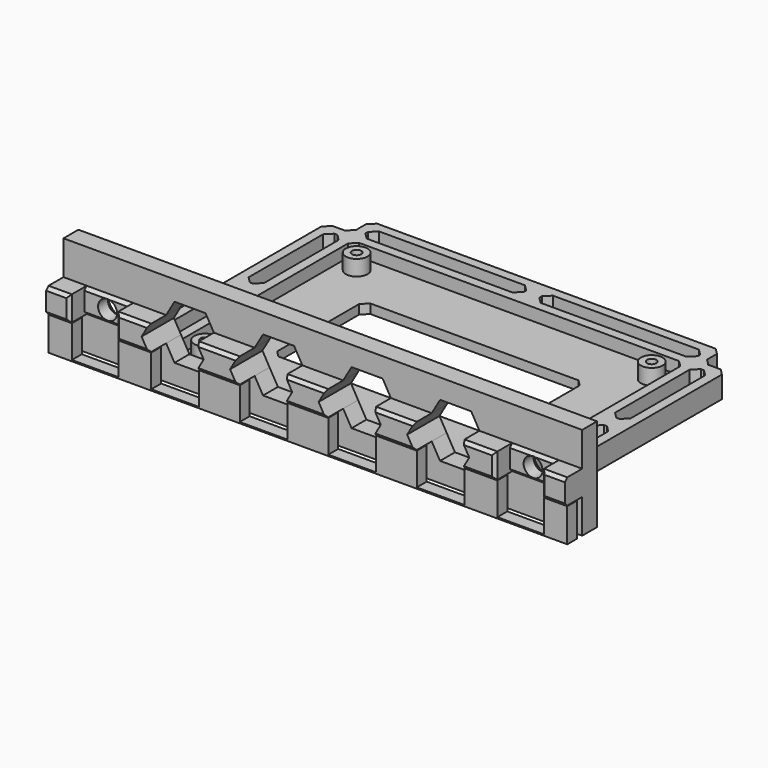
from build123d import *

# Parameters (mm, degrees)
F0_W          = 107
F0_H          = 73
F0_R          = 3.5
F0_W_2        = 71
F0_H_2        = 37
F0_R_2        = 1.5
F0_W_3        = 5
F0_H_3        = 5
F0_W_4        = 3
F0_H_4        = 3
F1_DEPTH      = 3
F2_DEPTH      = 4
F3_DEPTH      = 5
F4_DEPTH      = 27
F5_R          = 3.05
F6_DEPTH      = 6
F7_DEPTH      = 3
F5_W          = 7.5
F5_H          = 8
F8_DEPTH      = 7
F9_DEPTH      = 1
F10_T1_DEPTH  = 12.6433659759
F10_T3_DEPTH  = 15.7027670527
F10_T5_DEPTH  = 18.2621681294
F10_T7_DEPTH  = 18.2621681294
F10_T9_DEPTH  = 18.2621681294
F10_T11_DEPTH = 15.7027670527
F10_T13_DEPTH = 12.6433659759
F10_T15_DEPTH = 13.1433659759
F10_T20_DEPTH = 15
F10_T25_DEPTH = 15
F10_T30_DEPTH = 15
F10_T35_DEPTH = 15
F11_SIZE      = 2
F12_W         = 7.5
F12_H         = 4
F12_W_2       = 15
F12_W_3       = 10.5594010768
F12_W_4       = 15.3811978465
F12_W_5       = 13.1188021535
F13_DEPTH     = 0.4
F14_DEPTH     = 10.8


# Not quite as in the source:
# - a fillet or chamfer that OpenCascade refuses, or shapes differently, is made with other operations: its cross-section is extruded or revolved along the edge and cut away or added


with BuildPart() as f1:
    # F0 (on Top) → F1 (new body)
    with BuildSketch(Plane.XY):
        Rectangle(F0_W, F0_H)
        with Locations((-47.5, -30.5)):
            Circle(F0_R, mode=Mode.SUBTRACT)
        with Locations((47.5, -30.5)):
            Circle(F0_R, mode=Mode.SUBTRACT)
        Rectangle(F0_W_2, F0_H_2, mode=Mode.SUBTRACT)
        with Locations((-47.5, 30.5)):
            Circle(F0_R, mode=Mode.SUBTRACT)
        with Locations((47.5, 30.5)):
            Circle(F0_R, mode=Mode.SUBTRACT)
        with Locations((-47.5, 30.5)):
            Circle(F0_R)
        with Locations((-47.5, 30.5)):
            Circle(F0_R_2, mode=Mode.SUBTRACT)
        with Locations((-47.5, -30.5)):
            Circle(F0_R)
        with Locations((-47.5, -30.5)):
            Circle(F0_R_2, mode=Mode.SUBTRACT)
        with Locations((47.5, -30.5)):
            Circle(F0_R)
        with Locations((47.5, -30.5)):
            Circle(F0_R_2, mode=Mode.SUBTRACT)
        with Locations((47.5, 30.5)):
            Circle(F0_R)
        with Locations((47.5, 30.5)):
            Circle(F0_R_2, mode=Mode.SUBTRACT)
        Polygon((-53.5, -36.5), (-53.5, 36.5), (-56.5, 36.5), (-56.5, 2.5), (-56.5, -2.5), (-56.5, -36.5), align=None)
        Polygon((-56.5, 36.5), (-56.5, 39.5), (-64.5, 39.5), (-64.5, -36.5), (-61.5, -36.5), (-61.5, -2.5), (-61.5, 2.5), (-61.5, 36.5), align=None)
        with Locations((-59, 0)):
            Rectangle(F0_W_3, F0_H_3)
        with Locations((-55, 38)):
            Rectangle(F0_W_4, F0_H_4)
        Polygon((-53.5, 39.5), (-53.5, 44.5), (-2.5, 44.5), (2.5, 44.5), (53.5, 44.5), (53.5, 39.5), (56.5, 39.5), (56.5, 47.5), (-56.5, 47.5), (-56.5, 39.5), align=None)
        Polygon((-2.5, 39.5), (-53.5, 39.5), (-53.5, 36.5), (53.5, 36.5), (53.5, 39.5), (2.5, 39.5), align=None)
        Polygon((53.5, -36.5), (-53.5, -36.5), (-56.5, -36.5), (-61.5, -36.5), (-64.5, -36.5), (-83.5, -36.5), (-83.5, -42.5), (83.5, -42.5), (83.5, -36.5), (64.5, -36.5), (61.5, -36.5), (56.5, -36.5), align=None)
        with Locations((0, 42)):
            Rectangle(F0_W_3, F0_H_3)
        with Locations((55, 38)):
            Rectangle(F0_W_4, F0_H_4)
        Polygon((56.5, 39.5), (56.5, 36.5), (61.5, 36.5), (61.5, 2.5), (61.5, -2.5), (61.5, -36.5), (64.5, -36.5), (64.5, 39.5), align=None)
        with Locations((59, 0)):
            Rectangle(F0_W_3, F0_H_3)
        Polygon((56.5, 36.5), (53.5, 36.5), (53.5, -36.5), (56.5, -36.5), (56.5, -2.5), (56.5, 2.5), align=None)
    extrude(amount=-F1_DEPTH)

    # F0 (on Top) → F2 (join)
    with BuildSketch(Plane.XY):
        Polygon((-53.5, -36.5), (-53.5, 36.5), (-56.5, 36.5), (-56.5, 2.5), (-56.5, -2.5), (-56.5, -36.5), align=None)
        with Locations((-55, 38)):
            Rectangle(F0_W_4, F0_H_4)
        Polygon((-53.5, 39.5), (-53.5, 44.5), (-2.5, 44.5), (2.5, 44.5), (53.5, 44.5), (53.5, 39.5), (56.5, 39.5), (56.5, 47.5), (-56.5, 47.5), (-56.5, 39.5), align=None)
        Polygon((-56.5, 36.5), (-56.5, 39.5), (-64.5, 39.5), (-64.5, -36.5), (-61.5, -36.5), (-61.5, -2.5), (-61.5, 2.5), (-61.5, 36.5), align=None)
        with Locations((-59, 0)):
            Rectangle(F0_W_3, F0_H_3)
        with Locations((0, 42)):
            Rectangle(F0_W_3, F0_H_3)
        Polygon((-2.5, 39.5), (-53.5, 39.5), (-53.5, 36.5), (53.5, 36.5), (53.5, 39.5), (2.5, 39.5), align=None)
        with Locations((55, 38)):
            Rectangle(F0_W_4, F0_H_4)
        Polygon((56.5, 36.5), (53.5, 36.5), (53.5, -36.5), (56.5, -36.5), (56.5, -2.5), (56.5, 2.5), align=None)
        Polygon((56.5, 39.5), (56.5, 36.5), (61.5, 36.5), (61.5, 2.5), (61.5, -2.5), (61.5, -36.5), (64.5, -36.5), (64.5, 39.5), align=None)
        with Locations((59, 0)):
            Rectangle(F0_W_3, F0_H_3)
    extrude(amount=F2_DEPTH)

    # F0 (on Top) → F3 (join)
    with BuildSketch(Plane.XY):
        with Locations((-47.5, 30.5)):
            Circle(F0_R)
        with Locations((-47.5, 30.5)):
            Circle(F0_R_2, mode=Mode.SUBTRACT)
        with Locations((47.5, 30.5)):
            Circle(F0_R)
        with Locations((47.5, 30.5)):
            Circle(F0_R_2, mode=Mode.SUBTRACT)
        with Locations((47.5, -30.5)):
            Circle(F0_R)
        with Locations((47.5, -30.5)):
            Circle(F0_R_2, mode=Mode.SUBTRACT)
        with Locations((-47.5, -30.5)):
            Circle(F0_R)
        with Locations((-47.5, -30.5)):
            Circle(F0_R_2, mode=Mode.SUBTRACT)
    extrude(amount=F3_DEPTH)

    # F0 (on Top) → F4 (join)
    with BuildSketch(Plane.XY):
        Polygon((53.5, -36.5), (-53.5, -36.5), (-56.5, -36.5), (-61.5, -36.5), (-64.5, -36.5), (-83.5, -36.5), (-83.5, -42.5), (83.5, -42.5), (83.5, -36.5), (64.5, -36.5), (61.5, -36.5), (56.5, -36.5), align=None)
    extrude(amount=F4_DEPTH)

    # F5 (on face) → F6 (cut, through all)
    with BuildSketch(Plane.XZ.offset(42.5)):
        with BuildLine():
            ThreePointArc((-64.5808164115, 16), (-68.5, 17.6), (-72.4191835885, 16))
            Line((-72.4191835885, 16), (-64.5808164115, 16))
        make_face()
        with BuildLine():
            Line((-64.5808164115, 8), (-72.4191835885, 8))
            ThreePointArc((-72.4191835885, 8), (-68.5, 6.4), (-64.5808164115, 8))
        make_face()
        with BuildLine():
            Line((-64.5808164115, 16), (-72.4191835885, 16))
            ThreePointArc((-72.4191835885, 16), (-74.1, 12), (-72.4191835885, 8))
            Line((-72.4191835885, 8), (-64.5808164115, 8))
            ThreePointArc((-64.5808164115, 8), (-63.3372764893, 9.8306023987), (-62.9, 12))
            ThreePointArc((-62.9, 12), (-63.3372764893, 14.1693976013), (-64.5808164115, 16))
        make_face()
        with Locations((-68.5, 12)):
            Circle(F5_R, mode=Mode.SUBTRACT)
        with Locations((-68.5, 12)):
            Circle(F5_R)
        Polygon((-47.75, 20.6602540378), (-50.4405989232, 16), (-35.0594010768, 16), (-37.75, 20.6602540378), align=None)
        Polygon((-35.0594010768, 16), (-50.4405989232, 16), (-52.75, 12), (-50.4405989232, 8), (-35.0594010768, 8), (-32.75, 12), align=None)
        Polygon((-35.0594010768, 8), (-50.4405989232, 8), (-47.75, 3.3397459622), (-37.75, 3.3397459622), align=None)
        Polygon((-6.5594010768, 8), (-21.9405989232, 8), (-19.25, 3.3397459622), (-9.25, 3.3397459622), align=None)
        Polygon((-6.5594010768, 16), (-21.9405989232, 16), (-24.25, 12), (-21.9405989232, 8), (-6.5594010768, 8), (-4.25, 12), align=None)
        Polygon((-19.25, 20.6602540378), (-21.9405989232, 16), (-6.5594010768, 16), (-9.25, 20.6602540378), align=None)
        Polygon((9.25, 20.6602540378), (6.5594010768, 16), (21.9405989232, 16), (19.25, 20.6602540378), align=None)
        Polygon((21.9405989232, 16), (6.5594010768, 16), (4.25, 12), (6.5594010768, 8), (21.9405989232, 8), (24.25, 12), align=None)
        Polygon((21.9405989232, 8), (6.5594010768, 8), (9.25, 3.3397459622), (19.25, 3.3397459622), align=None)
        Polygon((47.75, 3.3397459622), (50.4405989232, 8), (35.0594010768, 8), (37.75, 3.3397459622), align=None)
        Polygon((52.75, 12), (50.4405989232, 16), (35.0594010768, 16), (32.75, 12), (35.0594010768, 8), (50.4405989232, 8), align=None)
        Polygon((35.0594010768, 16), (50.4405989232, 16), (47.75, 20.6602540378), (37.75, 20.6602540378), align=None)
        with BuildLine():
            Line((64.5808164115, 16), (72.4191835885, 16))
            ThreePointArc((72.4191835885, 16), (68.5, 17.6), (64.5808164115, 16))
        make_face()
        with BuildLine():
            ThreePointArc((74.1, 12), (73.6627235107, 14.1693976013), (72.4191835885, 16))
            Line((72.4191835885, 16), (64.5808164115, 16))
            ThreePointArc((64.5808164115, 16), (62.9, 12), (64.5808164115, 8))
            Line((64.5808164115, 8), (72.4191835885, 8))
            ThreePointArc((72.4191835885, 8), (73.6627235107, 9.8306023987), (74.1, 12))
        make_face()
        with Locations((68.5, 12)):
            Circle(F5_R, mode=Mode.SUBTRACT)
        with BuildLine():
            ThreePointArc((64.5808164115, 8), (68.5, 6.4), (72.4191835885, 8))
            Line((72.4191835885, 8), (64.5808164115, 8))
        make_face()
        with Locations((68.5, 12)):
            Circle(F5_R)
    extrude(amount=-F6_DEPTH, mode=Mode.SUBTRACT)

    # F5 (on face) → F7 (join, through all)
    with BuildSketch(Plane.XZ.offset(42.5)):
        with BuildLine():
            ThreePointArc((-64.5808164115, 16), (-68.5, 17.6), (-72.4191835885, 16))
            Line((-72.4191835885, 16), (-64.5808164115, 16))
        make_face()
        with BuildLine():
            Line((-64.5808164115, 16), (-72.4191835885, 16))
            ThreePointArc((-72.4191835885, 16), (-74.1, 12), (-72.4191835885, 8))
            Line((-72.4191835885, 8), (-64.5808164115, 8))
            ThreePointArc((-64.5808164115, 8), (-63.3372764893, 9.8306023987), (-62.9, 12))
            ThreePointArc((-62.9, 12), (-63.3372764893, 14.1693976013), (-64.5808164115, 16))
        make_face()
        with Locations((-68.5, 12)):
            Circle(F5_R, mode=Mode.SUBTRACT)
        with BuildLine():
            Line((-64.5808164115, 8), (-72.4191835885, 8))
            ThreePointArc((-72.4191835885, 8), (-68.5, 6.4), (-64.5808164115, 8))
        make_face()
        with BuildLine():
            ThreePointArc((64.5808164115, 8), (68.5, 6.4), (72.4191835885, 8))
            Line((72.4191835885, 8), (64.5808164115, 8))
        make_face()
        with BuildLine():
            ThreePointArc((74.1, 12), (73.6627235107, 14.1693976013), (72.4191835885, 16))
            Line((72.4191835885, 16), (64.5808164115, 16))
            ThreePointArc((64.5808164115, 16), (62.9, 12), (64.5808164115, 8))
            Line((64.5808164115, 8), (72.4191835885, 8))
            ThreePointArc((72.4191835885, 8), (73.6627235107, 9.8306023987), (74.1, 12))
        make_face()
        with Locations((68.5, 12)):
            Circle(F5_R, mode=Mode.SUBTRACT)
        with BuildLine():
            Line((64.5808164115, 16), (72.4191835885, 16))
            ThreePointArc((72.4191835885, 16), (68.5, 17.6), (64.5808164115, 16))
        make_face()
    extrude(amount=-F7_DEPTH)

    # F5 (on face) → F8 (join)
    with BuildSketch(Plane.XZ.offset(42.5)):
        with Locations((-79.75, 12)):
            Rectangle(F5_W, F5_H)
        with Locations((79.75, 12)):
            Rectangle(F5_W, F5_H)
        Polygon((61, 8), (61, 16), (50.4405989232, 16), (52.75, 12), (50.4405989232, 8), align=None)
        Polygon((32.75, 12), (35.0594010768, 16), (21.9405989232, 16), (24.25, 12), (21.9405989232, 8), (35.0594010768, 8), align=None)
        Polygon((6.5594010768, 16), (-6.5594010768, 16), (-4.25, 12), (-6.5594010768, 8), (6.5594010768, 8), (4.25, 12), align=None)
        Polygon((-21.9405989232, 16), (-35.0594010768, 16), (-32.75, 12), (-35.0594010768, 8), (-21.9405989232, 8), (-24.25, 12), align=None)
        Polygon((-50.4405989232, 16), (-61, 16), (-61, 8), (-50.4405989232, 8), (-52.75, 12), align=None)
    extrude(amount=F8_DEPTH)

    # F5 (on face) → F9 (join)
    with BuildSketch(Plane.XZ.offset(42.5)):
        with BuildLine():
            Line((-64.5808164115, 16), (-72.4191835885, 16))
            ThreePointArc((-72.4191835885, 16), (-74.1, 12), (-72.4191835885, 8))
            Line((-72.4191835885, 8), (-64.5808164115, 8))
            ThreePointArc((-64.5808164115, 8), (-63.3372764893, 9.8306023987), (-62.9, 12))
            ThreePointArc((-62.9, 12), (-63.3372764893, 14.1693976013), (-64.5808164115, 16))
        make_face()
        with Locations((-68.5, 12)):
            Circle(F5_R, mode=Mode.SUBTRACT)
        with BuildLine():
            Line((-61, 16), (-64.5808164115, 16))
            ThreePointArc((-64.5808164115, 16), (-63.3372764893, 14.1693976013), (-62.9, 12))
            ThreePointArc((-62.9, 12), (-63.3372764893, 9.8306023987), (-64.5808164115, 8))
            Line((-64.5808164115, 8), (-61, 8))
            Line((-61, 8), (-61, 16))
        make_face()
        with BuildLine():
            Line((-72.4191835885, 16), (-76, 16))
            Line((-76, 16), (-76, 8))
            Line((-76, 8), (-72.4191835885, 8))
            ThreePointArc((-72.4191835885, 8), (-74.1, 12), (-72.4191835885, 16))
        make_face()
        with BuildLine():
            ThreePointArc((64.5808164115, 8), (62.9, 12), (64.5808164115, 16))
            Line((64.5808164115, 16), (61, 16))
            Line((61, 16), (61, 8))
            Line((61, 8), (64.5808164115, 8))
        make_face()
        with BuildLine():
            ThreePointArc((74.1, 12), (73.6627235107, 14.1693976013), (72.4191835885, 16))
            Line((72.4191835885, 16), (64.5808164115, 16))
            ThreePointArc((64.5808164115, 16), (62.9, 12), (64.5808164115, 8))
            Line((64.5808164115, 8), (72.4191835885, 8))
            ThreePointArc((72.4191835885, 8), (73.6627235107, 9.8306023987), (74.1, 12))
        make_face()
        with Locations((68.5, 12)):
            Circle(F5_R, mode=Mode.SUBTRACT)
        with BuildLine():
            Line((76, 8), (76, 16))
            Line((76, 16), (72.4191835885, 16))
            ThreePointArc((72.4191835885, 16), (73.6627235107, 14.1693976013), (74.1, 12))
            ThreePointArc((74.1, 12), (73.6627235107, 9.8306023987), (72.4191835885, 8))
            Line((72.4191835885, 8), (76, 8))
        make_face()
    extrude(amount=F9_DEPTH)

    # F10: chamfer of 1 on 22 edges, made by hand

    # F10_s2 → F10_t1 (cut)
    with BuildSketch(Plane.YZ.offset(-86.071682988)):
        Polygon((-48.5, 8), (-49.5, 9), (-49.5, 8), align=None)
        Polygon((-49.5, 15), (-48.5, 16), (-49.5, 16), align=None)
    extrude(amount=F10_T1_DEPTH, mode=Mode.SUBTRACT)

    # F10_s4 → F10_t3 (cut)
    with BuildSketch(Plane.YZ.offset(-63.571682988)):
        Polygon((-48.5, 8), (-49.5, 9), (-49.5, 8), align=None)
        Polygon((-48.5, 16), (-49.5, 15), (-49.5, 16), align=None)
    extrude(amount=F10_T3_DEPTH, mode=Mode.SUBTRACT)

    # F10_s6 → F10_t5 (cut)
    with BuildSketch(Plane.YZ.offset(-37.6310840647)):
        Polygon((-48.5, 16), (-49.5, 15), (-49.5, 16), align=None)
        Polygon((-48.5, 8), (-49.5, 9), (-49.5, 8), align=None)
    extrude(amount=F10_T5_DEPTH, mode=Mode.SUBTRACT)

    # F10_s8 → F10_t7 (cut)
    with BuildSketch(Plane.YZ.offset(-9.1310840647)):
        Polygon((-48.5, 8), (-49.5, 9), (-49.5, 8), align=None)
        Polygon((-48.5, 16), (-49.5, 15), (-49.5, 16), align=None)
    extrude(amount=F10_T7_DEPTH, mode=Mode.SUBTRACT)

    # F10_s10 → F10_t9 (cut)
    with BuildSketch(Plane.YZ.offset(19.3689159353)):
        Polygon((-48.5, 16), (-49.5, 15), (-49.5, 16), align=None)
        Polygon((-48.5, 8), (-49.5, 9), (-49.5, 8), align=None)
    extrude(amount=F10_T9_DEPTH, mode=Mode.SUBTRACT)

    # F10_s12 → F10_t11 (cut)
    with BuildSketch(Plane.YZ.offset(47.8689159353)):
        Polygon((-48.5, 8), (-49.5, 9), (-49.5, 8), align=None)
        Polygon((-48.5, 16), (-49.5, 15), (-49.5, 16), align=None)
    extrude(amount=F10_T11_DEPTH, mode=Mode.SUBTRACT)

    # F10_s14 → F10_t13 (cut)
    with BuildSketch(Plane.YZ.offset(73.428317012)):
        Polygon((-48.5, 8), (-49.5, 9), (-49.5, 8), align=None)
        Polygon((-48.5, 16), (-49.5, 15), (-49.5, 16), align=None)
    extrude(amount=F10_T13_DEPTH, mode=Mode.SUBTRACT)

    # F10_s16 → F10_t15 (cut)
    with BuildSketch(Plane.XY.offset(5.428317012)):
        Polygon((-77, -49.5), (-76, -48.5), (-76, -49.5), align=None)
        Polygon((-61, -48.5), (-60, -49.5), (-61, -49.5), align=None)
        Polygon((61, -48.5), (60, -49.5), (61, -49.5), align=None)
        Polygon((77, -49.5), (76, -48.5), (76, -49.5), align=None)
    extrude(amount=F10_T15_DEPTH, mode=Mode.SUBTRACT)


with BuildPart() as f10_tool18:
    # F10_s19 → F10_t20 (new body)
    with BuildSketch(Plane.YZ.offset(-61)):
        Polygon((-42.5, 16), (-43.5, 15), (-43.5, 16), align=None)
    extrude(amount=-F10_T20_DEPTH)

    split(bisect_by=Plane.XZ.offset(42.5), keep=Keep.TOP)


with BuildPart() as f1_1:
    add(f1.part)

    # F10_t17: cut F10_tool18
    add(f10_tool18.part, mode=Mode.SUBTRACT)


with BuildPart() as f10_tool23:
    # F10_s24 → F10_t25 (new body)
    with BuildSketch(Plane.YZ.offset(-76)):
        Polygon((-42.5, 8), (-43.5, 9), (-43.5, 8), align=None)
    extrude(amount=F10_T25_DEPTH)

    split(bisect_by=Plane.XZ.offset(42.5), keep=Keep.TOP)


with BuildPart() as f1_2:
    add(f1_1.part)

    # F10_t22: cut F10_tool23
    add(f10_tool23.part, mode=Mode.SUBTRACT)


with BuildPart() as f10_tool28:
    # F10_s29 → F10_t30 (new body)
    with BuildSketch(Plane.YZ.offset(76)):
        Polygon((-42.5, 16), (-43.5, 15), (-43.5, 16), align=None)
    extrude(amount=-F10_T30_DEPTH)

    split(bisect_by=Plane.XZ.offset(42.5), keep=Keep.TOP)


with BuildPart() as f1_3:
    add(f1_2.part)

    # F10_t27: cut F10_tool28
    add(f10_tool28.part, mode=Mode.SUBTRACT)


with BuildPart() as f10_tool33:
    # F10_s34 → F10_t35 (new body)
    with BuildSketch(Plane.YZ.offset(61)):
        Polygon((-42.5, 8), (-43.5, 9), (-43.5, 8), align=None)
    extrude(amount=F10_T35_DEPTH)

    split(bisect_by=Plane.XZ.offset(42.5), keep=Keep.TOP)


with BuildPart() as f1_4:
    add(f1_3.part)

    # F10_t32: cut F10_tool33
    add(f10_tool33.part, mode=Mode.SUBTRACT)

    # F11
    f11_edges = [f1_4.edges().sort_by_distance(p)[0] for p in [
        (35.5, 18.5, -1.5),
        (35.5, -18.5, -1.5),
        (-35.5, 18.5, -1.5),
        (-35.5, -18.5, -1.5),
        (53.5, -36.5, 2),
        (61.5, -36.5, 0.5),
        (53.5, 36.5, 2),
        (61.5, 36.5, 0.5),
        (53.5, 44.5, 0.5),
        (56.5, 36.5, 0.5),
        (2.5, 44.5, 0.5),
        (56.5, -2.5, 0.5),
        (56.5, -36.5, 0.5),
        (56.5, 2.5, 0.5),
        (61.5, 2.5, 0.5),
        (53.5, 39.5, 0.5),
        (2.5, 39.5, 0.5),
        (-2.5, 44.5, 0.5),
        (-56.5, 36.5, 0.5),
        (-56.5, -2.5, 0.5),
        (-61.5, -2.5, 0.5),
        (-61.5, 36.5, 0.5),
        (-53.5, 44.5, 0.5),
        (-53.5, 39.5, 0.5),
        (-61.5, -36.5, 0.5),
        (-61.5, 2.5, 0.5),
        (-56.5, 2.5, 0.5),
        (-56.5, -36.5, 0.5),
        (-2.5, 39.5, 0.5),
        (-53.5, 36.5, 2),
        (-53.5, -36.5, 2),
        (64.5, 39.5, 0.5),
        (56.5, 47.5, 0.5),
        (56.5, 39.5, 0.5),
        (64.5, -36.5, 0.5),
        (-56.5, 47.5, 0.5),
        (-56.5, 39.5, 0.5),
        (-64.5, 39.5, 0.5),
        (-64.5, -36.5, 0.5),
        (61.5, -2.5, 0.5),
    ]]
    chamfer(f11_edges, length=F11_SIZE)


with BuildPart() as f13:
    # F12 (on face) → F13 (new body)
    with BuildSketch(Plane(origin=(0, 0, -3), x_dir=(1, 0, 0), z_dir=(0, 0, -1))):
        with Locations((-79.75, 46.5)):
            Rectangle(F12_W, F12_H)
        with Locations((-68.5, 46.5)):
            Rectangle(F12_W_2, F12_H)
        with Locations((-55.7202994616, 46.5)):
            Rectangle(F12_W_3, F12_H)
        with Locations((-42.75, 46.5)):
            Rectangle(F12_W_4, F12_H)
        with Locations((-28.5, 46.5)):
            Rectangle(F12_W_5, F12_H)
        with Locations((-14.25, 46.5)):
            Rectangle(F12_W_4, F12_H)
        with Locations((0, 46.5)):
            Rectangle(F12_W_5, F12_H)
        with Locations((14.25, 46.5)):
            Rectangle(F12_W_4, F12_H)
        with Locations((28.5, 46.5)):
            Rectangle(F12_W_5, F12_H)
        with Locations((42.75, 46.5)):
            Rectangle(F12_W_4, F12_H)
        with Locations((55.7202994616, 46.5)):
            Rectangle(F12_W_3, F12_H)
        with Locations((68.5, 46.5)):
            Rectangle(F12_W_2, F12_H)
        with Locations((79.75, 46.5)):
            Rectangle(F12_W, F12_H)
    extrude(amount=-F13_DEPTH)

    # F12 (on face) → F14 (join, through all)
    with BuildSketch(Plane(origin=(0, 0, -3), x_dir=(1, 0, 0), z_dir=(0, 0, -1))):
        with Locations((-79.75, 46.5)):
            Rectangle(F12_W, F12_H)
        with Locations((79.75, 46.5)):
            Rectangle(F12_W, F12_H)
        with Locations((-55.7202994616, 46.5)):
            Rectangle(F12_W_3, F12_H)
        with Locations((-28.5, 46.5)):
            Rectangle(F12_W_5, F12_H)
        with Locations((0, 46.5)):
            Rectangle(F12_W_5, F12_H)
        with Locations((28.5, 46.5)):
            Rectangle(F12_W_5, F12_H)
        with Locations((55.7202994616, 46.5)):
            Rectangle(F12_W_3, F12_H)
    extrude(amount=-F14_DEPTH)


solid = Compound([f1_4.part, f13.part])
